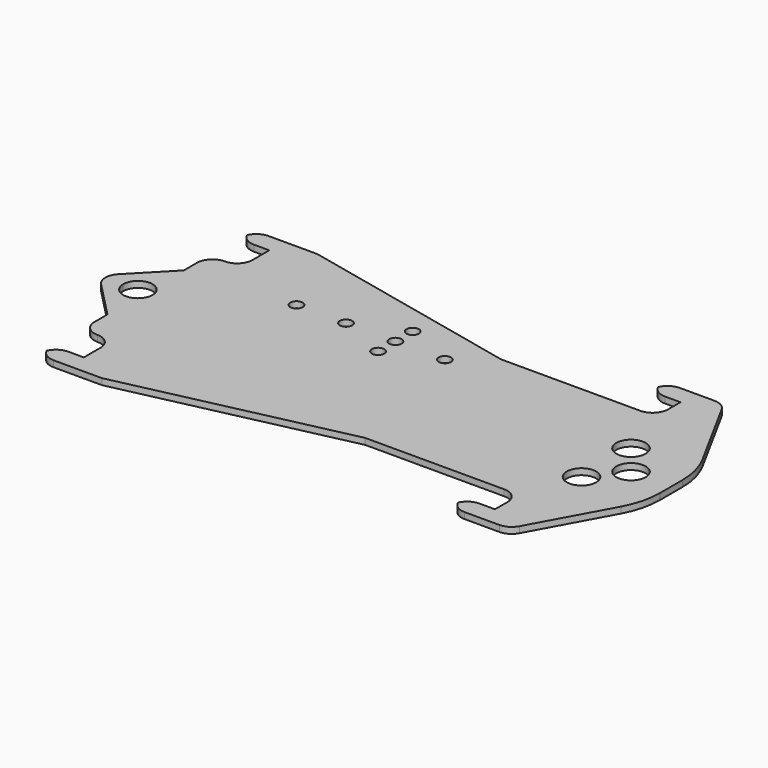
from build123d import *

# Parameters (mm, degrees)
F0_R        = 4.75
F0_R_2      = 2
F1_DEPTH    = 2
F2_T1_DEPTH = 16.8375789978
F2_T3_DEPTH = 27
F3_R        = 5
F4_R        = 4.99999
F5_R        = 25


# Not quite as in the source:
# - a fillet or chamfer that OpenCascade refuses, or shapes differently, is made with other operations: its cross-section is extruded or revolved along the edge and cut away or added
# - a fillet or chamfer is up to 0.001 mm smaller than in the source, because OpenCascade refuses the exact size


with BuildPart() as f1:
    # F0 (on Top) → F1 (new body)
    with BuildSketch(Plane.XY):
        Polygon((48, -43.5), (67.1863725781, -43.5), (85, -10.8566070522), (85, 10.8566070522), (67.1863725781, 43.5), (48, 43.5), (48, 37.5), (58, 37.5), (58, 27.5), (8, 27.5), (-64.2852836847, 43.5), (-85, 43.5), (-85, 37.5), (-75, 37.5), (-75, 25.7433671504), (-75, 0), (-75, -25.7433671504), (-75, -37.5), (-85, -37.5), (-85, -43.5), (-64.2852836847, -43.5), (8, -27.5), (58, -27.5), (58, -37.5), (48, -37.5), align=None)
        with Locations((64, -10)):
            Circle(F0_R, mode=Mode.SUBTRACT)
        with Locations((-51, 18.5)):
            Circle(F0_R_2, mode=Mode.SUBTRACT)
        with Locations((-35, 18.5)):
            Circle(F0_R_2, mode=Mode.SUBTRACT)
        with Locations((-19, 11.5)):
            Circle(F0_R_2, mode=Mode.SUBTRACT)
        with Locations((-19, 18.5)):
            Circle(F0_R_2, mode=Mode.SUBTRACT)
        with Locations((-19, 25.5)):
            Circle(F0_R_2, mode=Mode.SUBTRACT)
        with Locations((-3, 18.5)):
            Circle(F0_R_2, mode=Mode.SUBTRACT)
        with Locations((72, 0)):
            Circle(F0_R, mode=Mode.SUBTRACT)
        with Locations((64, 10)):
            Circle(F0_R, mode=Mode.SUBTRACT)
        with BuildLine():
            Line((-82.75, 0), (-75, 0))
            Line((-75, 0), (-75, 25.7433671504))
            Line((-75, 25.7433671504), (-85, 15.4460202903))
            Line((-85, 15.4460202903), (-85, 4.0388736054))
            ThreePointArc((-85, 4.0388736054), (-83.3504518318, 2.3116552511), (-82.75, 0))
        make_face()
        with BuildLine():
            Line((-85, 15.4460202903), (-100, 0))
            Line((-100, 0), (-92.25, 0))
            ThreePointArc((-92.25, 0), (-89.8116552511, 4.1495481682), (-85, 4.0388736054))
            Line((-85, 4.0388736054), (-85, 15.4460202903))
        make_face()
        with BuildLine():
            Line((-85, -4.0388736054), (-85, -15.4460202903))
            Line((-85, -15.4460202903), (-75, -25.7433671504))
            Line((-75, -25.7433671504), (-75, 0))
            Line((-75, 0), (-82.75, 0))
            ThreePointArc((-82.75, 0), (-83.3504518318, -2.3116552511), (-85, -4.0388736054))
        make_face()
        with BuildLine():
            Line((-100, 0), (-85, -15.4460202903))
            Line((-85, -15.4460202903), (-85, -4.0388736054))
            ThreePointArc((-85, -4.0388736054), (-89.8116552511, -4.1495481682), (-92.25, 0))
            Line((-92.25, 0), (-100, 0))
        make_face()
        Polygon((-75, 25.7433671504), (-85, 25.7433671504), (-85, 15.4460202903), align=None)
        Polygon((-85, -15.4460202903), (-85, -25.7433671504), (-75, -25.7433671504), align=None)
    extrude(amount=F1_DEPTH)

    # F2: fillet of radius 5 on 10 edges, made by hand

    # F2_s2 → F2_t1 (cut)
    with BuildSketch(Plane.XY.offset(-7.4187894989)):
        with BuildLine():
            ThreePointArc((68.607874454, 40.8951041407), (66.7707657989, 42.7997395679), (64.2188567786, 43.5))
            Line((64.2188567786, 43.5), (67.1863725781, 43.5))
            Line((67.1863725781, 43.5), (68.607874454, 40.8951041407))
        make_face()
        with BuildLine():
            ThreePointArc((64.2188567786, -43.5), (66.7707657989, -42.7997395679), (68.607874454, -40.8951041407))
            Line((68.607874454, -40.8951041407), (67.1863725781, -43.5))
            Line((67.1863725781, -43.5), (64.2188567786, -43.5))
        make_face()
    extrude(amount=F2_T1_DEPTH, mode=Mode.SUBTRACT)

    # F2_s4 → F2_t3 (cut)
    with BuildSketch(Plane.XY.offset(-12.5)):
        with BuildLine():
            ThreePointArc((53, 43.5), (49.4644660941, 42.0355339059), (48, 38.5))
            Line((48, 38.5), (48, 43.5))
            Line((48, 43.5), (53, 43.5))
        make_face()
        with BuildLine():
            ThreePointArc((-85, -38.5), (-83.5355339059, -42.0355339059), (-80, -43.5))
            Line((-80, -43.5), (-85, -43.5))
            Line((-85, -43.5), (-85, -38.5))
        make_face()
        with BuildLine():
            ThreePointArc((-80, -37.5), (-83.5355339059, -38.9644660941), (-85, -42.5))
            Line((-85, -42.5), (-85, -37.5))
            Line((-85, -37.5), (-80, -37.5))
        make_face()
        with BuildLine():
            ThreePointArc((48, -38.5), (49.4644660941, -42.0355339059), (53, -43.5))
            Line((53, -43.5), (48, -43.5))
            Line((48, -43.5), (48, -38.5))
        make_face()
        with BuildLine():
            ThreePointArc((53, -37.5), (49.4644660941, -38.9644660941), (48, -42.5))
            Line((48, -42.5), (48, -37.5))
            Line((48, -37.5), (53, -37.5))
        make_face()
        with BuildLine():
            ThreePointArc((48, 42.5), (49.4644660941, 38.9644660941), (53, 37.5))
            Line((53, 37.5), (48, 37.5))
            Line((48, 37.5), (48, 42.5))
        make_face()
        with BuildLine():
            ThreePointArc((-85, 42.5), (-83.5355339059, 38.9644660941), (-80, 37.5))
            Line((-80, 37.5), (-85, 37.5))
            Line((-85, 37.5), (-85, 42.5))
        make_face()
        with BuildLine():
            ThreePointArc((-80, 43.5), (-83.5355339059, 42.0355339059), (-85, 38.5))
            Line((-85, 38.5), (-85, 43.5))
            Line((-85, 43.5), (-80, 43.5))
        make_face()
    extrude(amount=F2_T3_DEPTH, mode=Mode.SUBTRACT)

    # F3
    f3_edges = [f1.edges().sort_by_distance(p)[0] for p in [
        (58, -27.5, 1),
        (58, 27.5, 1),
    ]]
    fillet(f3_edges, radius=F3_R)

    # F4 (radius 5 in the source; OpenCascade refuses exactly that, so slightly less here)
    f4_edges = [f1.edges().sort_by_distance(p)[0] for p in [
        (-85, 25.743367, 1),
        (-85, -25.743367, 1),
        (-75, 25.743367, 1),
        (-75, -25.743367, 1),
        (-100, 0, 1),
    ]]
    fillet(f4_edges, radius=F4_R)

    # F5
    f5_edges = [f1.edges().sort_by_distance(p)[0] for p in [
        (85, -10.856607, 1),
        (85, 10.856607, 1),
    ]]
    fillet(f5_edges, radius=F5_R)


solid = f1.part
